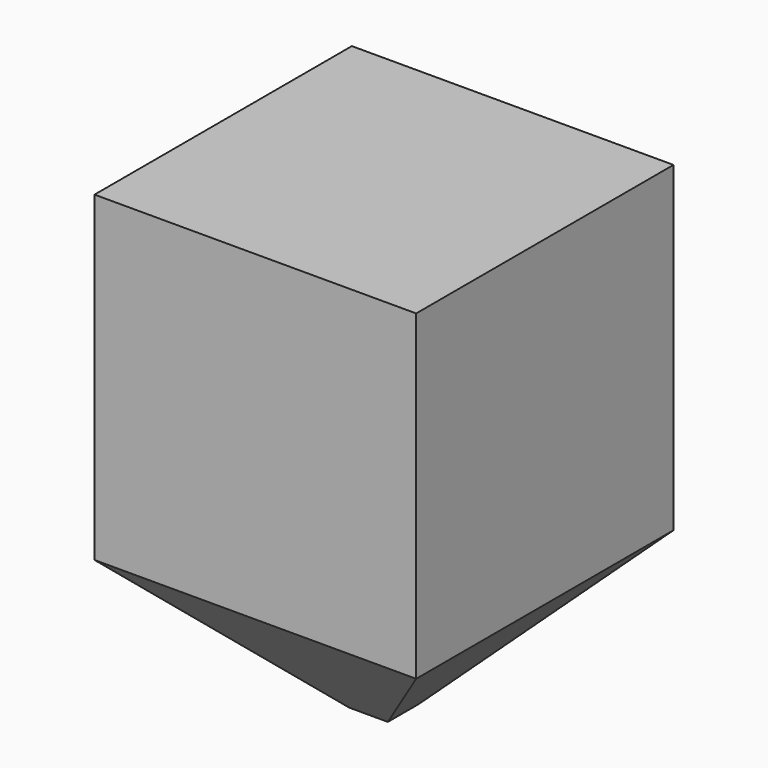
from build123d import *

# Parameters (mm, degrees)
F0_W          = 1000
F0_H          = 1000
F1_DEPTH      = 1000
F1_DEPTH_BACK = 440
F1_TAPER_BACK = 45


with BuildPart() as f1:
    # F0 (on Top) → F1 (new body, two sides)
    with BuildSketch(Plane.XY) as f1_sk:
        Rectangle(F0_W, F0_H)
    extrude(amount=F1_DEPTH)
    extrude(f1_sk.sketch, amount=-F1_DEPTH_BACK, taper=F1_TAPER_BACK)


solid = f1.part
